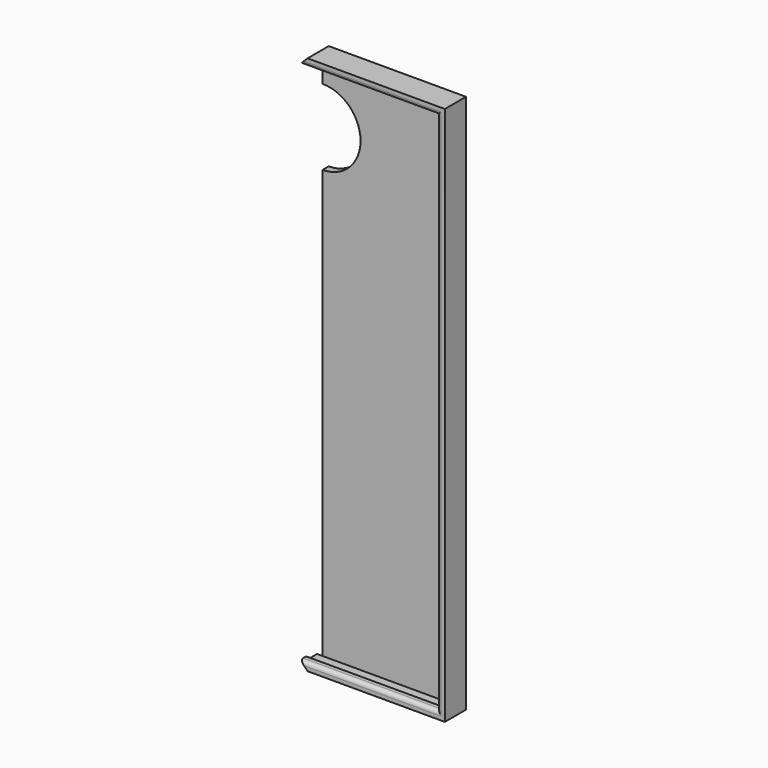
from build123d import *

# Parameters (mm, degrees)
F1_DEPTH = 6
F2_W     = 2
F2_H     = 142.7
F3_DEPTH = 24.3
F5_D     = 20
F7_DEPTH = 3
F9_DEPTH = 2
F10_R    = 1


# Not quite as in the source:
# - ends of sketch curves that miss each other by under 0.0002 mm in the source are joined


with BuildPart() as f1:
    # F0 (on Right) → F1 (new body, symmetric)
    with BuildSketch(Plane.YZ):
        Polygon((0.5, -10.3395825443), (0.5, 132.3604174557), (-0.5, 132.3604174557), (-0.5, 87.6604174557), (0, 87.6604174557), (0, 62.6604174557), (-0.5, 62.6604174557), (-0.5, 34.6604174557), (0, 34.6604174557), (0, 9.6604174557), (-0.5, 9.6604174557), (-0.5, -10.3395825443), align=None)
        Polygon((-0.5, 87.6604174557), (-0.5, 132.3604174557), (-1.5, 132.3604174557), (-1.5, -10.3395825443), (-0.5, -10.3395825443), (-0.5, 9.6604174557), (-1, 9.6604174557), (-1, 34.6604174557), (-0.5, 34.6604174557), (-0.5, 62.6604174557), (-1, 62.6604174557), (-1, 87.6604174557), align=None)
    extrude(amount=F1_DEPTH, both=True)

    # F2 (on face) → F3 (join)
    with BuildSketch(Plane.YZ.offset(6)):
        with Locations((-0.5, 61.0104174557)):
            Rectangle(F2_W, F2_H)
    extrude(amount=F3_DEPTH)

    # F5 (through all)
    with Locations(Plane.XZ.offset(1.5)):
        with Locations((-6, 114.3604174557)):
            Hole(F5_D / 2)

    # F6 (on face) → F7 (join)
    with BuildSketch(Plane.XZ.offset(1.5)):
        Polygon((30.3, 132.3604174557), (-6, 132.3604174557), (-7.5, 130.8604174557), (28.8, 130.8604174557), (28.8, -8.8395825443), (-7.5, -8.8395825443), (-6, -10.3395825443), (30.3, -10.3395825443), align=None)
    extrude(amount=F7_DEPTH)

    # F8 (on face) → F9 (join)
    with BuildSketch(Plane.XZ.offset(4.5)):
        Polygon((-6, -10.3395825443), (30.3, -10.3395825443), (30.3, 132.3604174557), (-6, 132.3604174557), (-8.0000020331, 130.3604154225), (28.3, 130.3604154225), (28.3, -8.3395825443), (-8, -8.3395825443), align=None)
    extrude(amount=F9_DEPTH)

    # F10
    f10_edges = [f1.edges().sort_by_distance(p)[0] for p in [
        (10.15, -6.5, -8.339583),
        (28.3, -6.5, 61.010416),
        (10.149999, -6.5, 130.360415),
    ]]
    fillet(f10_edges, radius=F10_R)


solid = f1.part
